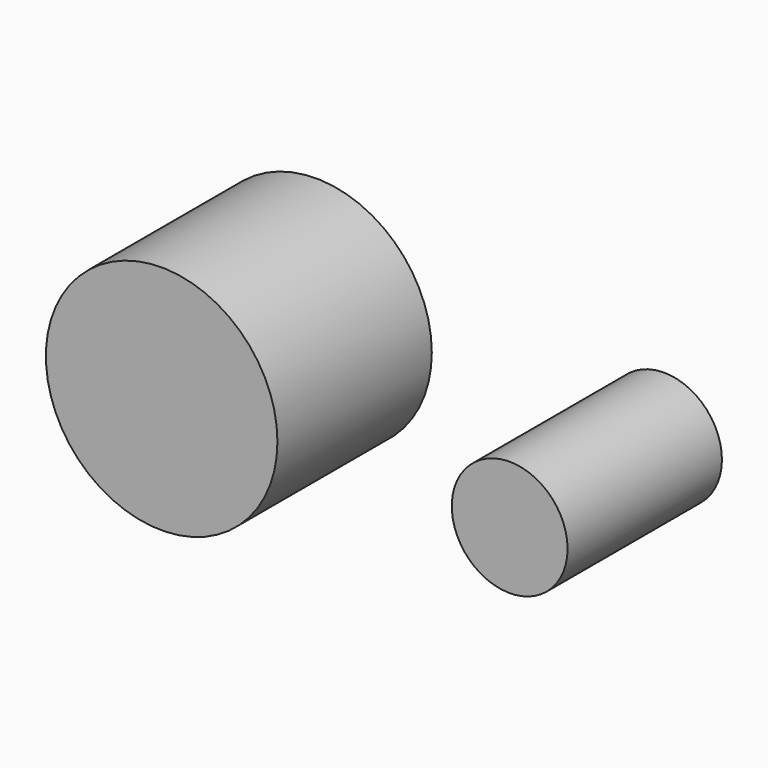
from build123d import *

# Parameters (mm, degrees)
F0_R     = 15
F1_DEPTH = 12.5
F0_R_2   = 7.5


# Not quite as in the source:
# - the program builds the solid bodies; features that only make, move or delete a surface that nothing else refers to are left out


with BuildPart() as f1:
    # F0 (on Front) → F1 (new body, symmetric)
    with BuildSketch(Plane.XZ):
        with Locations((37.3229645193, 25.7103565931)):
            Circle(F0_R)
    extrude(amount=F1_DEPTH, both=True)


with BuildPart() as f1b:
    # F0 (on Front) → F1, piece 2 (new body, symmetric)
    with BuildSketch(Plane.XZ):
        with Locations((82.4129134417, 25.7103565931)):
            Circle(F0_R_2)
    extrude(amount=F1_DEPTH, both=True)


solid = Compound([f1.part, f1b.part])
